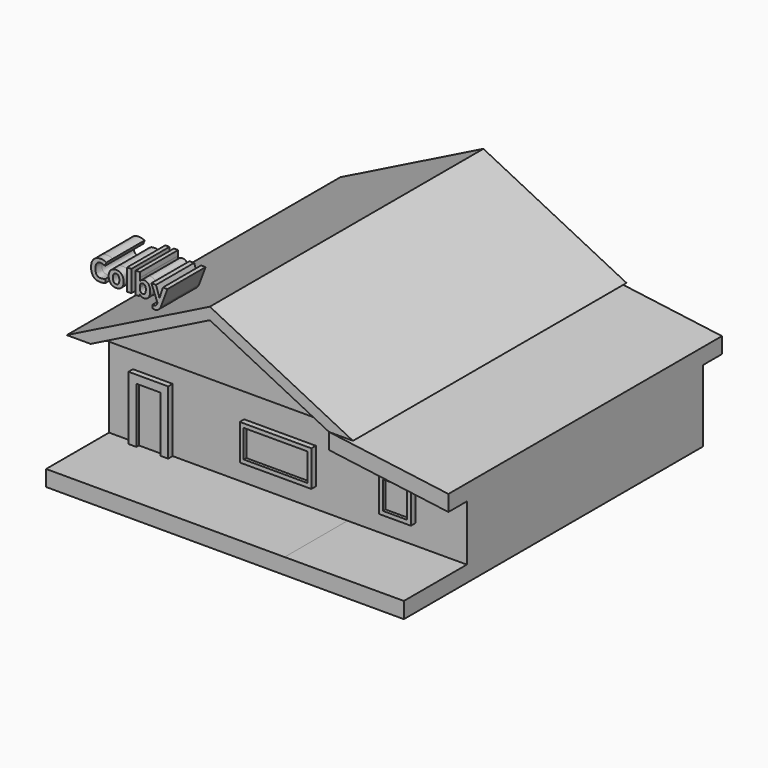
from build123d import *

# Parameters (mm, degrees)
F1_DEPTH       = 914.4
F1_DEPTH_BACK  = 12192
F0_W           = 2743.2
F0_H           = 1371.6
F0_W_2         = 1219.2
F0_W_3         = 2438.4
F0_H_2         = 1066.8
F0_W_4         = 914.4
F0_H_3         = 2133.6
F2_DEPTH       = 30.48
F2_DEPTH_BACK  = 11277.6
F3_DEPTH       = 3048
F3_DEPTH_BACK  = 11277.6
F4_DEPTH       = 457.2
F4_DEPTH_BACK  = 11734.8
F5_DEPTH       = 121.92
F6_DEPTH       = 243.84
F7_R           = 914.4
F7_R_2         = 762
F8_DEPTH       = 243.84
F9_DEPTH       = 121.92
F0_TEXT_SIZE   = 1082.5874076949
F10_DEPTH      = 304.8
F10_DEPTH_BACK = 1524


# Not quite as in the source:
# - Text() gives the source's letters only with a copy of the font that has no kerning and outlines rounded to 1/6400 em; it was checked with that copy


with BuildPart() as f1:
    # F0 (on Front) → F1 (new body, two sides)
    with BuildSketch(Plane.XZ) as f1_sk:
        Polygon((0, 2286), (4572, 0), (5486.4, 0), (0, 2743.2), align=None)
        Polygon((-5486.4, 0), (-4572, 0), (0, 2286), (0, 2743.2), align=None)
    extrude(amount=F1_DEPTH)
    extrude(f1_sk.sketch, amount=-F1_DEPTH_BACK)



with BuildPart() as f1b:
    # F0 (on Front) → F1, piece 2 (new body, two sides)
    with BuildSketch(Plane.XZ) as f1_2_sk:
        Polygon((9143.9956149355, -603.26778), (4572, 0), (4572, -609.6), (9143.9956149355, -1212.86778), align=None)
    extrude(amount=F1_DEPTH)
    extrude(f1_2_sk.sketch, amount=-F1_DEPTH_BACK)


with BuildPart() as f1_1:
    add(f1.part)

    add(f1b.part)  # F2 merges F1b
    # F0 (on Front) → F2 (join, two sides)
    with BuildSketch(Plane.XZ) as f2_sk:
        Polygon((4572, 0), (0, 0), (-4572, 0), (-4572, -3352.8), (-3657.6, -3352.8), (-3657.6, -914.4), (-2133.6, -914.4), (-2133.6, -3352.8), (4572, -3352.8), (4572, -609.6), align=None)
        with Locations((1981.2, -1905)):
            Rectangle(F0_W, F0_H, mode=Mode.SUBTRACT)
        Polygon((9143.9956149355, -1212.86778), (4572, -609.6), (4572, -3352.8), (9143.9956149355, -3346.46778), align=None)
        with Locations((6560.6431289673, -1905)):
            Rectangle(F0_W_2, F0_H, mode=Mode.SUBTRACT)
        with Locations((1981.2, -1905)):
            Rectangle(F0_W, F0_H)
        with Locations((1981.2, -1905)):
            Rectangle(F0_W_3, F0_H_2, mode=Mode.SUBTRACT)
        with Locations((1981.2, -1905)):
            Rectangle(F0_W_3, F0_H_2)
        with Locations((-2895.6, -2286)):
            Rectangle(F0_W_4, F0_H_3)
        Polygon((-3657.6, -914.4), (-3657.6, -3352.8), (-3352.8, -3352.8), (-3352.8, -1219.2), (-2438.4, -1219.2), (-2438.4, -3352.8), (-2133.6, -3352.8), (-2133.6, -914.4), align=None)
        with Locations((6560.6431289673, -1905)):
            Rectangle(F0_W_2, F0_H)
        with Locations((6560.6431289673, -1905)):
            Rectangle(F0_W_4, F0_H_2, mode=Mode.SUBTRACT)
        with Locations((6560.6431289673, -1905)):
            Rectangle(F0_W_4, F0_H_2)
    extrude(amount=F2_DEPTH)
    extrude(f2_sk.sketch, amount=-F2_DEPTH_BACK)

    # F0 (on Front) → F3 (join, two sides)
    with BuildSketch(Plane.XZ) as f3_sk:
        Polygon((-3657.6, -3352.8), (-4572, -3352.8), (-4572, -3962.4), (4572, -3962.4), (4572, -3352.8), (-2133.6, -3352.8), (-2438.4, -3352.8), (-3352.8, -3352.8), align=None)
        Polygon((9143.9956149355, -3346.46778), (4572, -3352.8), (4572, -3962.4), (9143.9956149355, -3962.4), align=None)
    extrude(amount=F3_DEPTH)
    extrude(f3_sk.sketch, amount=-F3_DEPTH_BACK)

    # F0 (on Front) → F5 (join)
    with BuildSketch(Plane.XZ):
        with Locations((-2895.6, -2286)):
            Rectangle(F0_W_4, F0_H_3)
        with Locations((1981.2, -1905)):
            Rectangle(F0_W_3, F0_H_2)
        with Locations((6560.6431289673, -1905)):
            Rectangle(F0_W_4, F0_H_2)
    extrude(amount=F5_DEPTH)

    # F0 (on Front) → F6 (join)
    with BuildSketch(Plane.XZ):
        Polygon((-3657.6, -914.4), (-3657.6, -3352.8), (-3352.8, -3352.8), (-3352.8, -1219.2), (-2438.4, -1219.2), (-2438.4, -3352.8), (-2133.6, -3352.8), (-2133.6, -914.4), align=None)
        with Locations((1981.2, -1905)):
            Rectangle(F0_W, F0_H)
        with Locations((1981.2, -1905)):
            Rectangle(F0_W_3, F0_H_2, mode=Mode.SUBTRACT)
        with Locations((6560.6431289673, -1905)):
            Rectangle(F0_W_2, F0_H)
        with Locations((6560.6431289673, -1905)):
            Rectangle(F0_W_4, F0_H_2, mode=Mode.SUBTRACT)
    extrude(amount=F6_DEPTH)

    # F7 (on face) → F8 (join)
    with BuildSketch(Plane(origin=(-4572, 0, 0), x_dir=(0, -1, 0), z_dir=(-1, 0, 0))):
        with Locations((-7623.1763792357, -1828.8)):
            Circle(F7_R)
        with Locations((-7623.1763792357, -1828.8)):
            Circle(F7_R_2, mode=Mode.SUBTRACT)
        Polygon((-2590.8, -754.6804338455), (-5062.9209756653, -754.6804338455), (-3826.8604878326, -2895.6), align=None)
        Polygon((-2854.7645430735, -907.0804338455), (-3826.8604878326, -2590.8), (-4798.9564325918, -907.0804338455), align=None, mode=Mode.SUBTRACT)
    extrude(amount=F8_DEPTH)

    # F7 (on face) → F9 (join)
    with BuildSketch(Plane(origin=(-4572, 0, 0), x_dir=(0, -1, 0), z_dir=(-1, 0, 0))):
        with Locations((-7623.1763792357, -1828.8)):
            Circle(F7_R_2)
        Polygon((-4798.9564325918, -907.0804338455), (-3826.8604878326, -2590.8), (-2854.7645430735, -907.0804338455), align=None)
    extrude(amount=F9_DEPTH)


with BuildPart() as f4:
    # F0 (on Front) → F4 (new body, two sides)
    with BuildSketch(Plane.XZ) as f4_sk:
        Polygon((-4572, 0), (0, 0), (0, 2286), align=None)
        Polygon((0, 2286), (0, 0), (4572, 0), align=None)
    extrude(amount=F4_DEPTH)
    extrude(f4_sk.sketch, amount=-F4_DEPTH_BACK)


with BuildPart() as f10:
    # F0 (on Front) → F10 (new body, two sides)
    with BuildSketch(Plane.XZ) as f10_sk:
        with Locations((-5105.1750183105, 1809.9828958511)):
            Text('Colby', F0_TEXT_SIZE, font='Open Sans', font_style=FontStyle.BOLD, text_align=(TextAlign.LEFT, TextAlign.BOTTOM))
    extrude(amount=F10_DEPTH)
    extrude(f10_sk.sketch, amount=-F10_DEPTH_BACK)


solid = Compound([f1_1.part, f4.part, f10.part])
